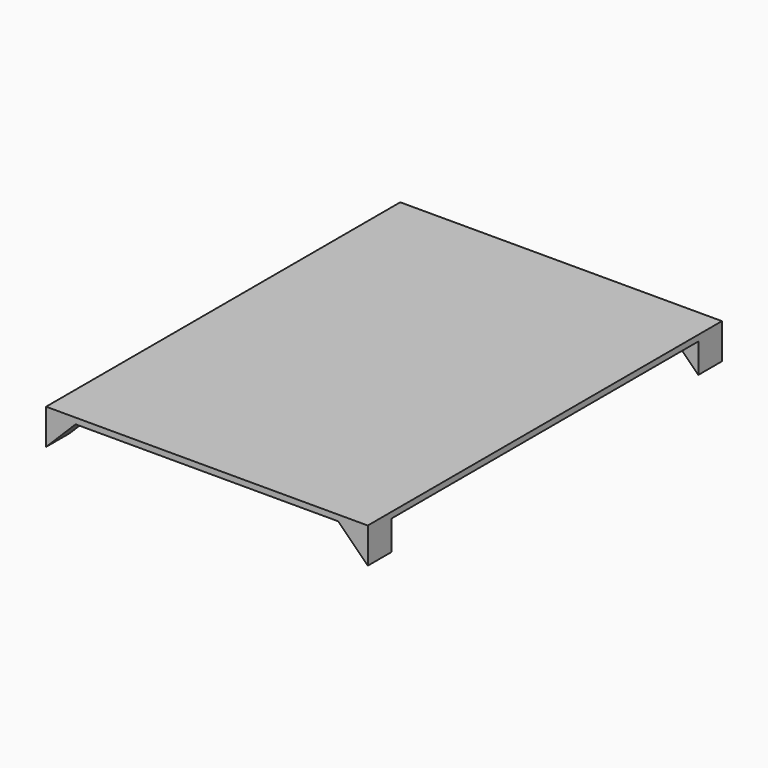
from build123d import *

# Parameters (mm, degrees)
F0_W     = 276.86
F0_H     = 5.08
F1_DEPTH = 381
F2_W     = 25.4
F2_H     = 25.4
F3_DEPTH = 25.4
F4_SIZE  = 25.39999
F5_SIZE  = 25.39999


# Not quite as in the source:
# - a fillet or chamfer is up to 0.001 mm smaller than in the source, because OpenCascade refuses the exact size


with BuildPart() as f1:
    # F0 (on Front) → F1 (new body)
    with BuildSketch(Plane.XZ):
        Rectangle(F0_W, F0_H)
    extrude(amount=F1_DEPTH)

    # F2 (on face) → F3 (join)
    with BuildSketch(Plane(origin=(0, 0, -2.54), x_dir=(1, 0, 0), z_dir=(0, 0, -1))):
        with Locations((125.73, 368.3)):
            Rectangle(F2_W, F2_H)
        with Locations((-125.73, 368.3)):
            Rectangle(F2_W, F2_H)
        with Locations((-125.73, 12.7)):
            Rectangle(F2_W, F2_H)
        with Locations((125.73, 12.7)):
            Rectangle(F2_W, F2_H)
    extrude(amount=F3_DEPTH)

    # F4 (size 25.4 in the source; OpenCascade refuses exactly that, so slightly less here)
    f4_edges = [f1.edges().sort_by_distance(p)[0] for p in [
        (-113.03, -368.3, -27.94),
    ]]
    chamfer(f4_edges, length=F4_SIZE)

    # F5 (size 25.4 in the source; OpenCascade refuses exactly that, so slightly less here)
    f5_edges = [f1.edges().sort_by_distance(p)[0] for p in [
        (113.03, -368.3, -27.94),
        (113.03, -12.7, -27.94),
        (-113.03, -12.7, -27.94),
    ]]
    chamfer(f5_edges, length=F5_SIZE)


solid = f1.part
